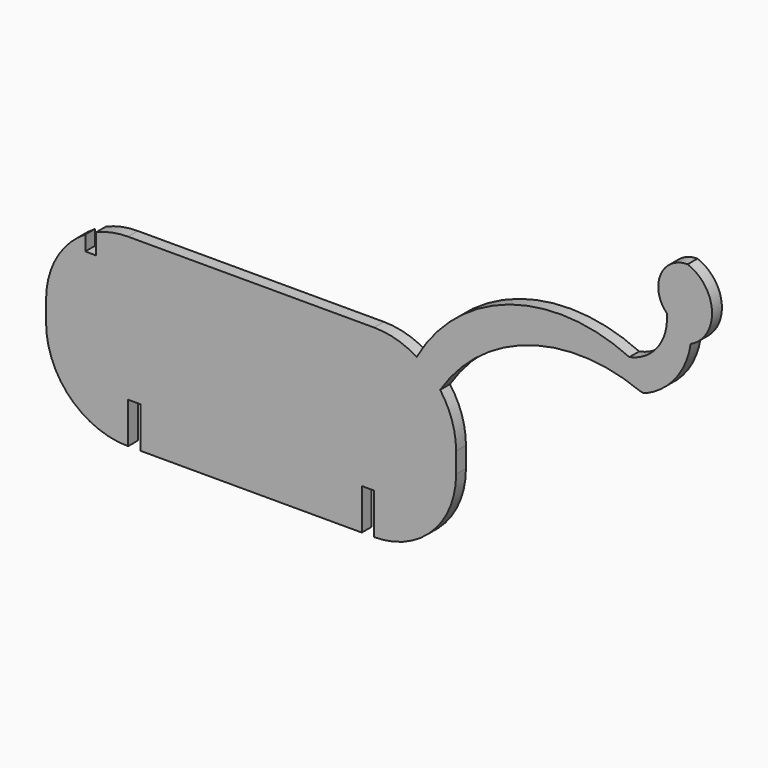
from build123d import *

# Parameters (mm, degrees)
F1_DEPTH = 3


# Not quite as in the source:
# - ends of sketch curves that miss each other by under 0.0002 mm in the source are joined


with BuildPart() as f1:
    # F0 (on Front) → F1 (new body)
    with BuildSketch(Plane.XZ):
        with BuildLine():
            Line((27.6752540097, 25.9776275605), (-32.3247459903, 25.9776275605))
            ThreePointArc((-32.3247459903, 25.9776275605), (-36.2904670893, 25.5805114342), (-40.0987030081, 24.4049331771))
            Line((-40.0987030081, 24.4049331771), (-40.0987030081, 19.4049331771))
            Line((-40.0987030081, 19.4049331771), (-42.7675568515, 19.4049331771))
            Line((-42.7675568515, 19.4049331771), (-42.7675568515, 23.0348166993))
            ThreePointArc((-42.7675568515, 23.0348166993), (-49.7726143017, 15.7537152948), (-52.3247459903, 5.9776275605))
            Line((-52.3247459903, 5.9776275605), (-52.3247459903, 0.9776275605))
            ThreePointArc((-52.3247459903, 0.9776275605), (-46.4668816141, -13.1645080632), (-32.3247459903, -19.0223724395))
            Line((-32.3247459903, -19.0223724395), (-32.3247459903, -9.0223724395))
            Line((-32.3247459903, -9.0223724395), (-29.3247459903, -9.0223724395))
            Line((-29.3247459903, -9.0223724395), (-29.3247459903, -19.0223724395))
            Line((-29.3247459903, -19.0223724395), (24.6752540097, -19.0223724395))
            Line((24.6752540097, -19.0223724395), (24.6752540097, -9.0223724395))
            Line((24.6752540097, -9.0223724395), (27.6752540097, -9.0223724395))
            Line((27.6752540097, -9.0223724395), (27.6752540097, -19.0223724395))
            ThreePointArc((27.6752540097, -19.0223724395), (41.8173896334, -13.1645080632), (47.6752540097, 0.9776275605))
            Line((47.6752540097, 0.9776275605), (47.6752540097, 5.9776275605))
            ThreePointArc((47.6752540097, 5.9776275605), (46.6766261397, 12.2184493954), (43.7804682921, 17.8360453688))
            ThreePointArc((43.7804682921, 17.8360453688), (65.3177378121, 34.4466284435), (92.4979172096, 33.4449816105))
            ThreePointArc((92.4979172096, 33.4449816105), (93.2694445512, 33.2995729147), (94.0374965073, 33.4623435853))
            ThreePointArc((94.0374965073, 33.4623435853), (101.2901547391, 39.0961583347), (104.8859376265, 47.5466769297))
            ThreePointArc((104.8859376265, 47.5466769297), (110.0970401084, 56.2336783381), (104.1383245347, 64.4259484991))
            ThreePointArc((104.1383245347, 64.4259484991), (97.5285801831, 60.0432380566), (99.0521934878, 52.2602133107))
            ThreePointArc((99.0521934878, 52.2602133107), (96.8833215141, 44.3091582137), (89.9362853313, 39.8749765827))
            ThreePointArc((89.9362853313, 39.8749765827), (60.6981355661, 41.6708405362), (38.0764996773, 23.060194363))
            ThreePointArc((38.0764996773, 23.060194363), (33.0765808814, 25.2344618804), (27.6752540097, 25.9776275605))
        make_face()
    extrude(amount=F1_DEPTH)


solid = f1.part
